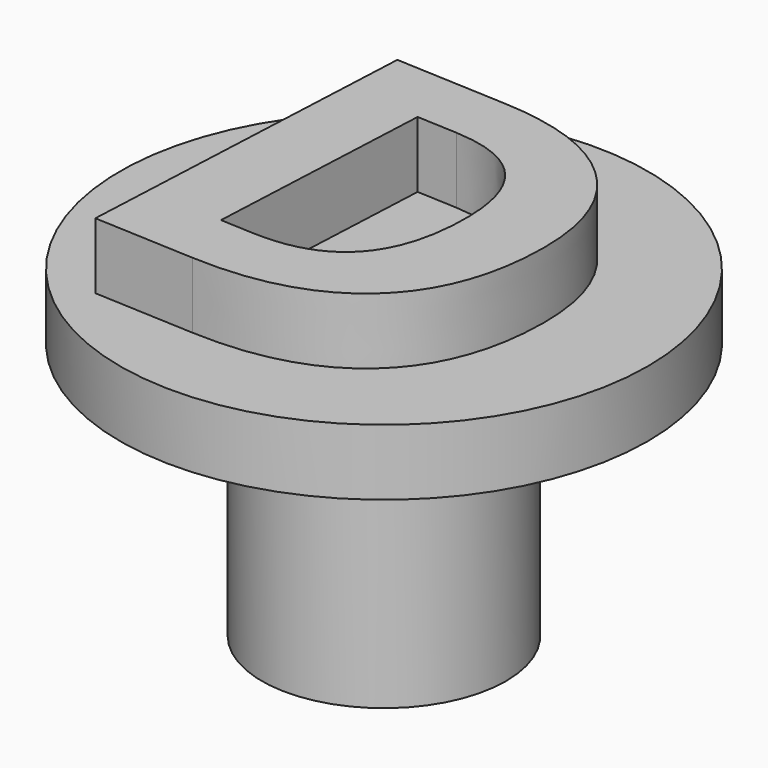
from build123d import *

# Parameters (mm, degrees)
F0_R         = 0.925
F1_DEPTH     = 1.95
F2_R         = 2
F3_DEPTH     = 0.5
F4_TEXT_SIZE = 3.7882939849
F5_DEPTH     = 0.5


# Not quite as in the source:
# - Text() gives the source's letters only with a copy of the font that has no kerning and outlines rounded to 1/6400 em; it was checked with that copy


with BuildPart() as f1:
    # F0 (on Top) → F1 (new body)
    with BuildSketch(Plane.XY):
        Circle(F0_R)
    extrude(amount=F1_DEPTH)

    # F2 (on face) → F3 (join)
    with BuildSketch(Plane.XY.offset(1.95)):
        Circle(F2_R)
    extrude(amount=F3_DEPTH)

    # F4 (on face) → F5 (join)
    with BuildSketch(Plane.XY.offset(2.45)):
        with Locations(Location((-1.4775757552, -1.2957121159), (0, 0, -2.6963058565))):
            Text('D', F4_TEXT_SIZE, font='Open Sans', font_style=FontStyle.BOLD, text_align=(TextAlign.LEFT, TextAlign.BOTTOM))
    extrude(amount=F5_DEPTH)


solid = f1.part
